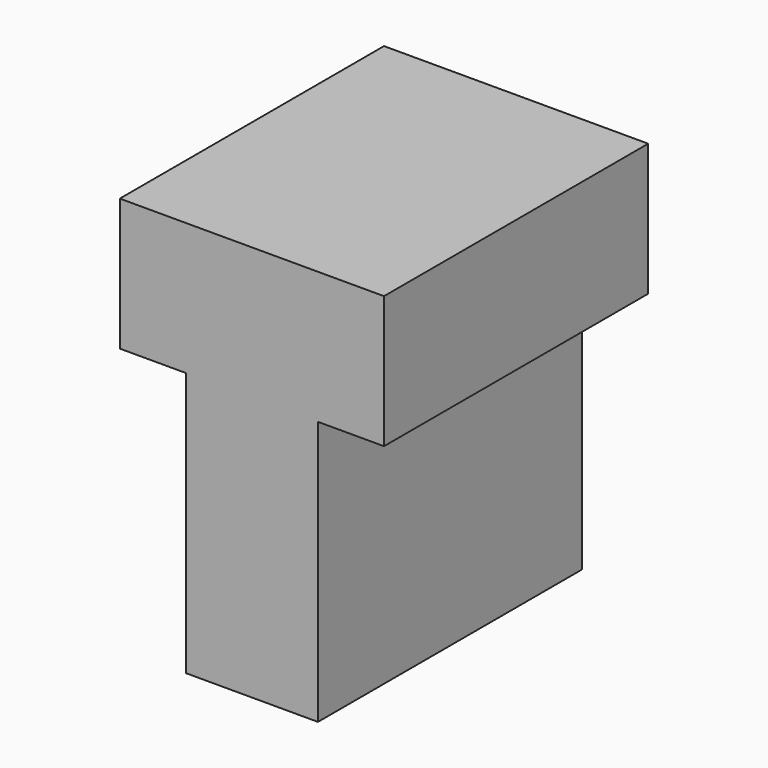
from build123d import *

# Parameters (mm, degrees)
F1_DEPTH = 31.75


# Not quite as in the source:
# - a length typed as a fraction of an inch, garbled in the dataset ("3 / 203.2 mm" for 3/8 in), is restored


with BuildPart() as f1:
    # F0 (on Front) → F1 (new body)
    with BuildSketch(Plane.XZ):
        Polygon((0, 0), (12.7, 0), (12.7, 25.4), (19.05, 25.4), (19.05, 38.1), (-6.35, 38.1), (-6.35, 25.4), (0, 25.4), align=None)
    extrude(amount=F1_DEPTH)


solid = f1.part
